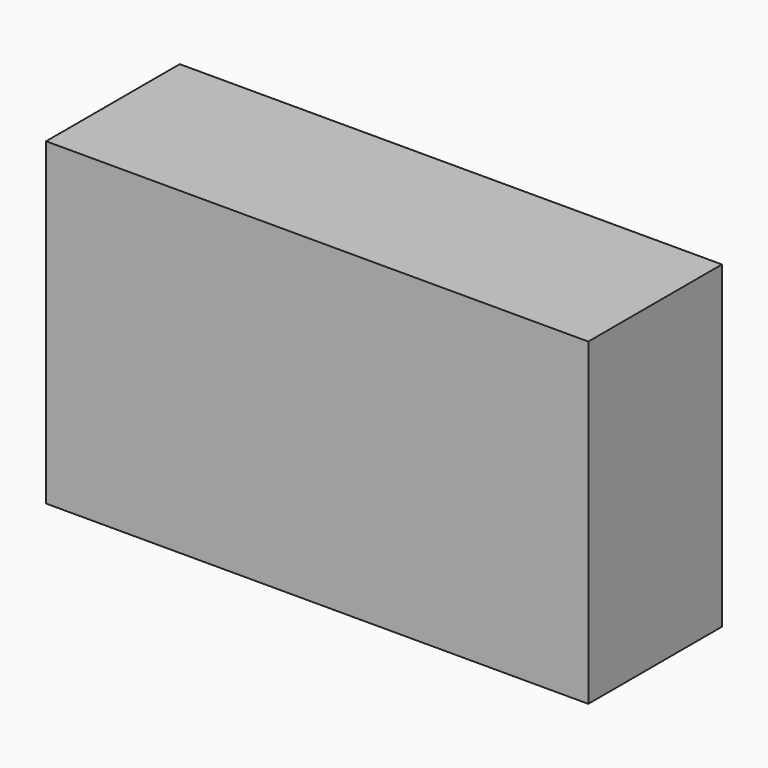
from build123d import *

# Parameters (mm, degrees)
F0_W     = 82.4639983475
F0_H     = 48.5082380474
F1_DEPTH = 25.4
F2_W     = 13.8226579875
F2_H     = 35.7262613252
F3_DEPTH = 5.08
F4_R     = 5.07999


# Not quite as in the source:
# - a fillet or chamfer is up to 0.001 mm smaller than in the source, because OpenCascade refuses the exact size


with BuildPart() as f1:
    # F0 (on Front) → F1 (new body)
    with BuildSketch(Plane.XZ):
        with Locations((4.3657366186, -4.1232034564)):
            Rectangle(F0_W, F0_H)
    extrude(amount=F1_DEPTH)

    # F2 (on face) → F3 (join)
    with BuildSketch(Plane(origin=(-36.8662625551, 0, 0), x_dir=(0, -1, 0), z_dir=(-1, 0, 0))):
        with Locations((12.4125434086, -4.4842208736)):
            Rectangle(F2_W, F2_H)
    extrude(amount=F3_DEPTH)

    # F4 (radius 5.08 in the source; OpenCascade refuses exactly that, so slightly less here)
    f4_edges = [f1.edges().sort_by_distance(p)[0] for p in [
        (-41.946263, -12.412543, -22.347352),
        (-41.946263, -5.501214, -4.484221),
        (-41.946263, -19.323872, -4.484221),
        (-41.946263, -12.412543, 13.37891),
    ]]
    fillet(f4_edges, radius=F4_R)


solid = f1.part
